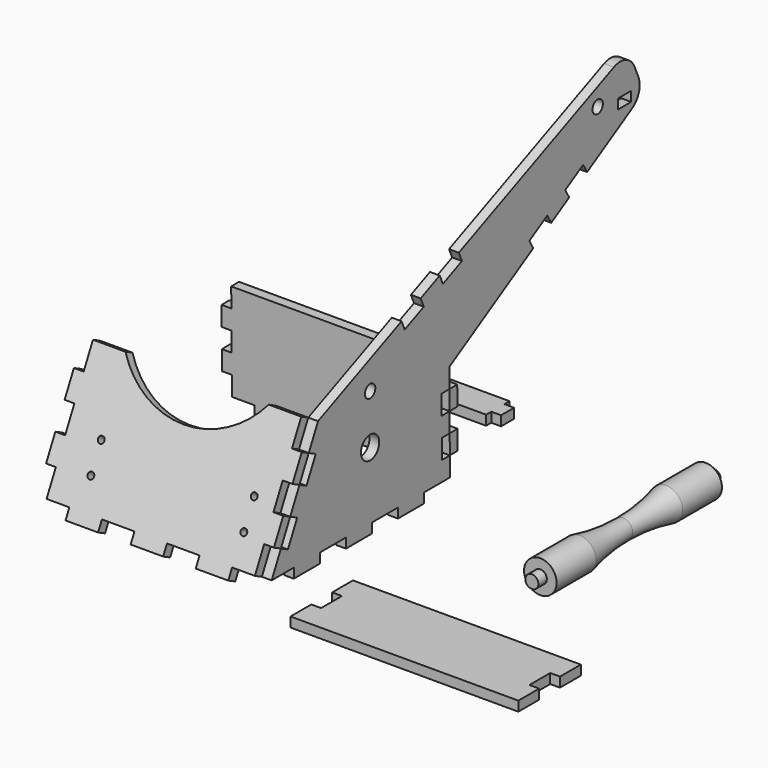
from build123d import *

# Parameters (mm, degrees)
F0_R      = 3.5
F0_R_2    = 2
F0_W      = 5
F0_H      = 3
F1_DEPTH  = 3
F2_R      = 1
F3_DEPTH  = 3
F5_DEPTH  = 3
F8_W      = 3
F8_H      = 5
F8_W_2    = 64
F8_H_2    = 2
F8_R      = 2.25
F9_DEPTH  = 3
F10_R     = 1.49999
F12_DEPTH = 3


# Not quite as in the source:
# - a fillet or chamfer is up to 0.001 mm smaller than in the source, because OpenCascade refuses the exact size


with BuildPart() as f1:
    # F0 (on Right) → F1 (new body)
    with BuildSketch(Plane.YZ):
        with BuildLine():
            Line((20, 0), (29.973435353, 0))
            Line((29.973435353, 0), (29.9203081417, 5.999764787))
            Line((29.9203081417, 5.999764787), (26.9204257482, 5.9732011814))
            Line((26.9204257482, 5.9732011814), (26.8672985369, 11.9729659684))
            Line((26.8672985369, 11.9729659684), (29.8671809304, 11.999529574))
            Line((29.8671809304, 11.999529574), (29.8140537191, 17.999294361))
            Line((29.8140537191, 17.999294361), (26.8141713256, 17.9727307554))
            Line((26.8141713256, 17.9727307554), (26.7610441143, 23.9724955424))
            Line((26.7610441143, 23.9724955424), (29.7609265078, 23.999059148))
            Line((29.7609265078, 23.999059148), (29.7077992965, 29.998823935))
            Line((29.7077992965, 29.998823935), (61.9676767232, 49.0069065975))
            Line((61.9676767232, 49.0069065975), (60.4447307691, 51.5915991558))
            Line((60.4447307691, 51.5915991558), (67.337244258, 55.6527883666))
            Line((67.337244258, 55.6527883666), (68.860190212, 53.0680958083))
            Line((68.860190212, 53.0680958083), (75.7527037009, 57.1292850192))
            Line((75.7527037009, 57.1292850192), (74.2297577468, 59.7139775775))
            Line((74.2297577468, 59.7139775775), (81.1222712357, 63.7751667883))
            Line((81.1222712357, 63.7751667883), (82.6452171897, 61.19047423))
            Line((82.6452171897, 61.19047423), (99.8765009118, 71.3434472571))
            ThreePointArc((99.8765009118, 71.3434472571), (102.5381164942, 74.6623302131), (102.330253897, 78.9115624643))
            Line((102.330253897, 78.9115624643), (100.8565268492, 82.2904234142))
            ThreePointArc((100.8565268492, 82.2904234142), (97.5495598407, 85.476687835), (92.9581518653, 85.3913382168))
            Line((92.9581518653, 85.3913382168), (33.3786655213, 59.4050955683))
            Line((33.3786655213, 59.4050955683), (34.5780305666, 56.6552731216))
            Line((34.5780305666, 56.6552731216), (27.2451707089, 53.4569663341))
            Line((27.2451707089, 53.4569663341), (26.0458056636, 56.2067887808))
            Line((26.0458056636, 56.2067887808), (18.7129458059, 53.0084819933))
            Line((18.7129458059, 53.0084819933), (19.9123108512, 50.2586595466))
            Line((19.9123108512, 50.2586595466), (12.5794509935, 47.0603527591))
            Line((12.5794509935, 47.0603527591), (11.3800859481, 49.8101752057))
            Line((11.3800859481, 49.8101752057), (-20.7011759294, 35.8175830104))
            Line((-20.7011759294, 35.8175830104), (-24.2626405006, 28.6540664083))
            Line((-24.2626405006, 28.6540664083), (-21.5763217748, 27.3185171941))
            Line((-21.5763217748, 27.3185171941), (-25.137786346, 20.155000592))
            Line((-25.137786346, 20.155000592), (-27.8241050717, 21.4905498062))
            Line((-27.8241050717, 21.4905498062), (-31.3855696429, 14.3270332041))
            Line((-31.3855696429, 14.3270332041), (-28.6992509171, 12.99148399))
            Line((-28.6992509171, 12.99148399), (-32.2607154883, 5.8279673879))
            Line((-32.2607154883, 5.8279673879), (-34.9470342141, 7.1635166021))
            Line((-34.9470342141, 7.1635166021), (-38.5084987853, 0))
            Line((-38.5084987853, 0), (-30, 0))
            Line((-30, 0), (-30, -3))
            Line((-30, -3), (-20, -3))
            Line((-20, -3), (-20, 0))
            Line((-20, 0), (-10, 0))
            Line((-10, 0), (-10, -3))
            Line((-10, -3), (0, -3))
            Line((0, -3), (0, 0))
            Line((0, 0), (10, 0))
            Line((10, 0), (10, -3))
            Line((10, -3), (20, -3))
            Line((20, -3), (20, 0))
        make_face()
        with Locations((-0.7011764626, 20.5706802606)):
            Circle(F0_R, mode=Mode.SUBTRACT)
        with Locations((-0.7011764626, 35.8129646274)):
            Circle(F0_R_2, mode=Mode.SUBTRACT)
        with Locations((86.7076262675, 77.2102056698)):
            Circle(F0_R_2, mode=Mode.SUBTRACT)
        with Locations((97.0504930615, 74.791040957)):
            Rectangle(F0_W, F0_H, mode=Mode.SUBTRACT)
    extrude(amount=F1_DEPTH)


with BuildPart() as f3:
    # F2 (on face) → F3 (new body)
    with BuildSketch(Plane(origin=(0, -30.8765776965, 15.3508177134), x_dir=(1, 0, 0), z_dir=(0, -0.8954395753, 0.4451830714))):
        with BuildLine():
            Line((0, 21.1145205949), (0, 22.8566682358))
            Line((0, 22.8566682358), (-10, 22.8566682358))
            ThreePointArc((-10, 22.8566682358), (-32, 11.2296143244), (-54, 22.8566682358))
            Line((-54, 22.8566682358), (-64, 22.8566682358))
            Line((-64, 22.8566682358), (-64, 19.6977295541))
            Line((-64, 19.6977295541), (-64, 14.8566682358))
            Line((-64, 14.8566682358), (-67, 14.8566682358))
            Line((-67, 14.8566682358), (-67, 6.8566682358))
            Line((-67, 6.8566682358), (-64, 6.8566682358))
            Line((-64, 6.8566682358), (-64, -1.1433317642))
            Line((-64, -1.1433317642), (-67, -1.1433317642))
            Line((-67, -1.1433317642), (-67, -9.1433317642))
            Line((-67, -9.1433317642), (-64, -9.1433317642))
            Line((-64, -9.1433317642), (-64, -17.1433317642))
            Line((-64, -17.1433317642), (-57, -17.1433317642))
            Line((-57, -17.1433317642), (-57, -20.4433317642))
            Line((-57, -20.4433317642), (-47, -20.4433317642))
            Line((-47, -20.4433317642), (-47, -17.1433317642))
            Line((-47, -17.1433317642), (-37, -17.1433317642))
            Line((-37, -17.1433317642), (-37, -20.4433317642))
            Line((-37, -20.4433317642), (-27, -20.4433317642))
            Line((-27, -20.4433317642), (-27, -17.1433317642))
            Line((-27, -17.1433317642), (-17, -17.1433317642))
            Line((-17, -17.1433317642), (-17, -20.4433317642))
            Line((-17, -20.4433317642), (-7, -20.4433317642))
            Line((-7, -20.4433317642), (-7, -17.1433317642))
            Line((-7, -17.1433317642), (0, -17.1433317642))
            Line((0, -17.1433317642), (0, -9.1433317642))
            Line((0, -9.1433317642), (3, -9.1433317642))
            Line((3, -9.1433317642), (3, -1.1433317642))
            Line((3, -1.1433317642), (0, -1.1433317642))
            Line((0, -1.1433317642), (0, 6.8566682358))
            Line((0, 6.8566682358), (3, 6.8566682358))
            Line((3, 6.8566682358), (3, 14.8566682358))
            Line((3, 14.8566682358), (0, 14.8566682358))
            Line((0, 14.8566682358), (0, 21.1145205949))
        make_face()
        with Locations((-53.6014225595, -8.1433317642)):
            Circle(F2_R, mode=Mode.SUBTRACT)
        with Locations((-53.6014225595, 0.8566682358)):
            Circle(F2_R, mode=Mode.SUBTRACT)
        with Locations((-6.6014225595, -8.1433317642)):
            Circle(F2_R, mode=Mode.SUBTRACT)
        with Locations((-6.6014225595, 0.8566682358)):
            Circle(F2_R, mode=Mode.SUBTRACT)
    extrude(amount=F3_DEPTH)


with BuildPart() as f5:
    # F4 (on face) → F5 (new body)
    with BuildSketch(Plane(origin=(0, 29.9710853519, 0.2653904346), x_dir=(-1, 0, 0), z_dir=(0, 0.9999607978, 0.0088545352))):
        Polygon((64, 29.7345991611), (0, 29.7345991611), (0, 23.7345991611), (-3, 23.7345991611), (-3, 17.7345991611), (0, 17.7345991611), (0, 11.7345991611), (-3, 11.7345991611), (-3, 5.7345991611), (0, 5.7345991611), (0, -0.2654008389), (7, -0.2654008389), (7, -3.3154008389), (17, -3.3154008389), (17, -0.2654008389), (27, -0.2654008389), (27, -3.3154008389), (37, -3.3154008389), (37, -0.2654008389), (47, -0.2654008389), (47, -3.3154008389), (57, -3.3154008389), (57, -0.2654008389), (64, -0.2654008389), (64, 5.7345991611), (67, 5.7345991611), (67, 11.7345991611), (64, 11.7345991611), (64, 17.7345991611), (67, 17.7345991611), (67, 23.7345991611), (64, 23.7345991611), align=None)
    extrude(amount=F5_DEPTH)


with BuildPart() as f7:
    # F6 (on Top) → F7 (revolve)
    with BuildSketch(Plane.XY):
        with BuildLine():
            Line((50.1375770867, 0), (52.1375770867, 0))
            Line((52.1375770867, 0), (52.1375770867, 70))
            Line((52.1375770867, 70), (50.1375770867, 70))
            Line((50.1375770867, 70), (50.1375770867, 66.75))
            Line((50.1375770867, 66.75), (47.1375770867, 66.75))
            Line((47.1375770867, 66.75), (47.1375770867, 51.6132477258))
            ThreePointArc((47.1375770867, 51.6132477258), (48.6357785023, 43.3666002653), (49.1375770867, 35))
            ThreePointArc((49.1375770867, 35), (48.6357785023, 26.6333997347), (47.1375770867, 18.3867522742))
            Line((47.1375770867, 18.3867522742), (47.1375770867, 3.25))
            Line((47.1375770867, 3.25), (50.1375770867, 3.25))
            Line((50.1375770867, 3.25), (50.1375770867, 0))
        make_face()
    revolve(axis=Axis((52.1375770867, 35, 0), (0, 1, 0)))


with BuildPart() as f9:
    # F8 (on Top) → F9 (new body)
    with BuildSketch(Plane.XY):
        with Locations((-5.5079954267, 60.8603270352)):
            Rectangle(F8_W, F8_H)
        with Locations((-72.5079954267, 60.8603270352)):
            Rectangle(F8_W, F8_H)
        with Locations((-39.0079954267, 57.3603270352)):
            Rectangle(F8_W_2, F8_H_2)
        with Locations((-39.0079954267, 60.8603270352)):
            Rectangle(F8_W_2, F8_H)
        with Locations((-39.0079954267, 60.8603270352)):
            Circle(F8_R, mode=Mode.SUBTRACT)
        with Locations((-39.0079954267, 64.3603270352)):
            Rectangle(F8_W_2, F8_H_2)
    extrude(amount=F9_DEPTH)

    # F10 (radius 1.5 in the source; OpenCascade refuses exactly that, so slightly less here)
    f10_edges = [f9.edges().sort_by_distance(p)[0] for p in [
        (-41.257995, 60.860327, 3),
        (-41.257995, 60.860327, 0),
    ]]
    fillet(f10_edges, radius=F10_R)


with BuildPart() as f12:
    # F11 (on Top) → F12 (new body)
    with BuildSketch(Plane.XY):
        Polygon((91.834442392, -38.8147931695), (91.834442392, -30.8147931695), (21.834442392, -30.8147931695), (21.834442392, -38.8147931695), (24.834442392, -38.8147931695), (24.834442392, -46.8147931695), (21.834442392, -46.8147931695), (21.834442392, -54.8147931695), (91.834442392, -54.8147931695), (91.834442392, -46.8147931695), (88.834442392, -46.8147931695), (88.834442392, -38.8147931695), align=None)
    extrude(amount=F12_DEPTH)


solid = Compound([f1.part, f3.part, f5.part, f7.part, f9.part, f12.part])
